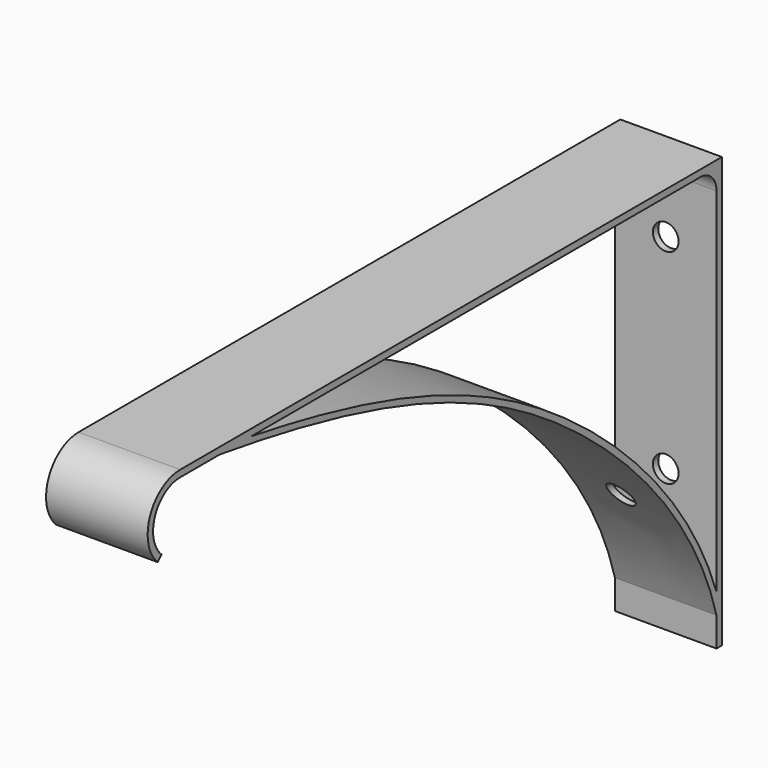
from build123d import *

# Parameters (mm, degrees)
F0_W      = 15
F0_H      = 63.5
F1_DEPTH  = 1
F2_W      = 15
F2_H      = 100
F3_DEPTH  = 1
F5_DEPTH  = 15
F7_D      = 3.7973
F7_DEPTH  = 1.0010001
F8_D      = 3.7973
F8_DEPTH  = 99.0010001
F9_D      = 3.7973
F10_R     = 3
F12_DEPTH = 15


# Not quite as in the source:
# - the dataset's text gives a spline's control points without its knots; the knots are read off the source's solid


with BuildPart() as f1:
    # F0 (on Front) → F1 (new body)
    with BuildSketch(Plane.XZ):
        with Locations((0, -31.75)):
            Rectangle(F0_W, F0_H)
    extrude(amount=F1_DEPTH)

    # F2 (on Top) → F3 (join)
    with BuildSketch(Plane.XY):
        with Locations((0, -50)):
            Rectangle(F2_W, F2_H)
    extrude(amount=-F3_DEPTH)

    # F4 (on face) → F5 (join, through all)
    with BuildSketch(Plane.YZ.offset(7.5)):
        with BuildLine():
            add(Edge.make_bspline(
                [(-1, -59.1678209603), (-4.7628395259, -45.3067980707), (-29.7762758586, -17.4602950514), (-61.8860200047, -5.5842199363), (-92.6793441176, -1)],
                knots=[0, 0, 0, 0, 0.4491979362, 1, 1, 1, 1], degree=3))
            Line((-1, -59.1678209603), (-0.1314357545, -58.9320325989))
            add(Edge.make_bspline(
                [(-0.1314357545, -58.9320325989), (-1.2015793269, -54.989987117), (-3.6884016693, -49.2559925066), (-8.3530917512, -42.083257521), (-12.4261382193, -36.9661666224), (-16.9750747913, -32.1385398724), (-21.9011436861, -27.6279890298), (-27.1107997825, -23.4618046647), (-32.4934625877, -19.6712415186), (-38.1217352473, -16.235966274), (-44.0944999552, -13.1322911599), (-50.5030405646, -10.3365734857), (-59.7536135039, -6.9863101985), (-72.8745679903, -3.4418665365), (-85.5418056788, -1.1526510188), (-92.5468210682, -0.109810334)],
                knots=[0, 0, 0, 0, 0.125, 0.1875, 0.25, 0.3125, 0.375, 0.4375, 0.5, 0.5625, 0.625, 0.6875, 0.75, 0.875, 1, 1, 1, 1], degree=3))
            Line((-92.5468210682, -0.109810334), (-92.6793441176, -1))
        make_face()
    extrude(amount=-F5_DEPTH)

    # F7 (through all, one way)
    with BuildSketch(Plane.XZ.offset(1)):
        with Locations((0, -12.3973852023)):
            Circle(F7_D / 2)
    extrude(amount=-F7_DEPTH, mode=Mode.SUBTRACT)

    # F8 (through all, one way)
    with BuildSketch(Plane(origin=(0, -1, 0), x_dir=(1, 0, 0), z_dir=(0, 1, 0))):
        with Locations((0, 42.5568334758)):
            Circle(F8_D / 2)
    extrude(amount=-F8_DEPTH, mode=Mode.SUBTRACT)

    # F9 (through all)
    with Locations(Plane.XZ.offset(1)):
        with Locations((0, -42.5568334758)):
            Hole(F9_D / 2)

    # F10
    f10_edges = [f1.edges().sort_by_distance(p)[0] for p in [
        (0, -1, -1),
    ]]
    fillet(f10_edges, radius=F10_R)

    # F11 (on face) → F12 (join, through all)
    with BuildSketch(Plane.YZ.offset(7.5)):
        with BuildLine():
            Line((-100, -1), (-100, 0))
            ThreePointArc((-100, 0), (-105.5726686693, -3.7761825834), (-104.1308658813, -10.3515453659))
            Line((-104.1308658813, -10.3515453659), (-103.4423882344, -9.6262878049))
            ThreePointArc((-103.4423882344, -9.6262878049), (-104.6438905577, -4.1468188195), (-100, -1))
        make_face()
    extrude(amount=-F12_DEPTH)


solid = f1.part
